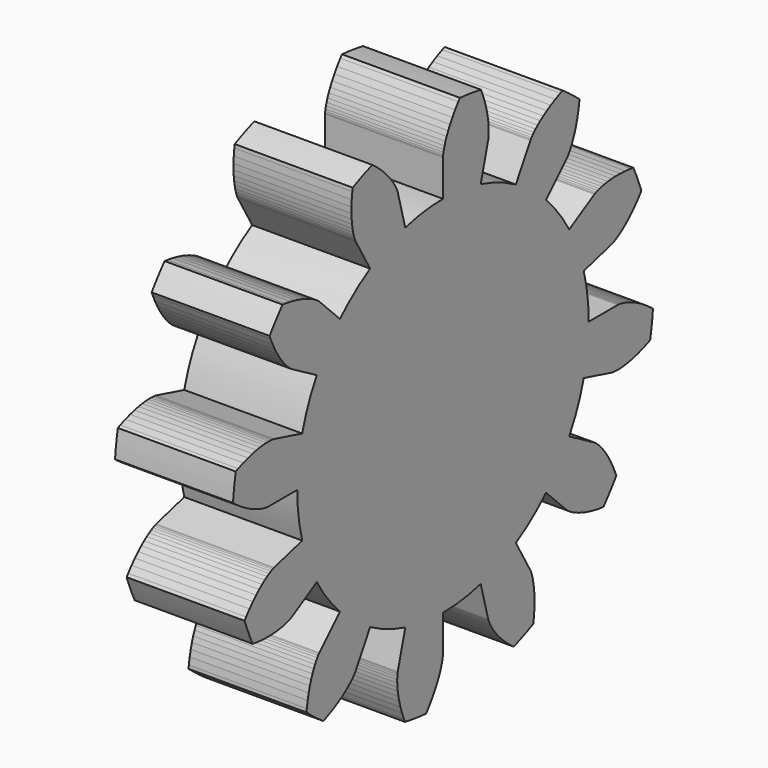
from build123d import *

# Parameters (mm, degrees)
F2_DEPTH = 4.9784


# Not quite as in the source:
# - a variable given as a bare number and used for a length is read in inches; the dataset says mm whatever the document's units were
# - a feature names something its author has since deleted; it is built from what else it names


with BuildPart() as f2:
    # F1 (on Right) → F2 (new body)
    with BuildSketch(Plane.YZ):
        with BuildLine():
            ThreePointArc((7.426291308, -1.9898687587), (7.6224883485, -1.0035196289), (7.6882625, 0))
            ThreePointArc((7.6882625, 0), (7.6224883485, 1.0035196289), (7.426291308, 1.9898687587))
            ThreePointArc((7.426291308, 1.9898687587), (7.1030283643, 2.9421706824), (6.658230636, 3.84413125))
            ThreePointArc((6.658230636, 3.84413125), (6.0995087354, 4.6803176661), (5.4364225493, 5.4364225493))
            ThreePointArc((5.4364225493, 5.4364225493), (4.6803176661, 6.0995087354), (3.84413125, 6.658230636))
            ThreePointArc((3.84413125, 6.658230636), (2.9421706824, 7.1030283643), (1.9898687587, 7.426291308))
            ThreePointArc((1.9898687587, 7.426291308), (1.0035196289, 7.6224883485), (0, 7.6882625))
            ThreePointArc((0, 7.6882625), (-1.0035196289, 7.6224883485), (-1.9898687587, 7.426291308))
            ThreePointArc((-1.9898687587, 7.426291308), (-2.9421706824, 7.1030283643), (-3.84413125, 6.658230636))
            ThreePointArc((-3.84413125, 6.658230636), (-4.6803176661, 6.0995087354), (-5.4364225493, 5.4364225493))
            ThreePointArc((-5.4364225493, 5.4364225493), (-6.0995087354, 4.6803176661), (-6.658230636, 3.84413125))
            ThreePointArc((-6.658230636, 3.84413125), (-7.1030283643, 2.9421706824), (-7.426291308, 1.9898687587))
            ThreePointArc((-7.426291308, 1.9898687587), (-7.6224883485, 1.0035196289), (-7.6882625, 0))
            ThreePointArc((-7.6882625, 0), (-7.6224883485, -1.0035196289), (-7.426291308, -1.9898687587))
            ThreePointArc((-7.426291308, -1.9898687587), (-7.1030283643, -2.9421706824), (-6.658230636, -3.84413125))
            ThreePointArc((-6.658230636, -3.84413125), (-6.0995087354, -4.6803176661), (-5.4364225493, -5.4364225493))
            ThreePointArc((-5.4364225493, -5.4364225493), (-4.6803176661, -6.0995087354), (-3.84413125, -6.658230636))
            ThreePointArc((-3.84413125, -6.658230636), (-2.9421706824, -7.1030283643), (-1.9898687587, -7.426291308))
            ThreePointArc((-1.9898687587, -7.426291308), (-1.0035196289, -7.6224883485), (0, -7.6882625))
            ThreePointArc((0, -7.6882625), (1.0035196289, -7.6224883485), (1.9898687587, -7.426291308))
            ThreePointArc((1.9898687587, -7.426291308), (2.9421706824, -7.1030283643), (3.84413125, -6.658230636))
            ThreePointArc((3.84413125, -6.658230636), (4.6803176661, -6.0995087354), (5.4364225493, -5.4364225493))
            ThreePointArc((5.4364225493, -5.4364225493), (6.0995087354, -4.6803176661), (6.658230636, -3.84413125))
            ThreePointArc((6.658230636, -3.84413125), (7.1030283643, -2.9421706824), (7.426291308, -1.9898687587))
        make_face()
        with BuildLine():
            Line((-7.9861452975, -4.6108031373), (-6.658230636, -3.84413125))
            ThreePointArc((-6.658230636, -3.84413125), (-7.1030283643, -2.9421706824), (-7.426291308, -1.9898687587))
            Line((-7.426291308, -1.9898687587), (-8.9073876605, -2.3867273303))
            Line((-8.9073876605, -2.3867273303), (-8.9184155168, -2.3900799169))
            Line((-8.9184155168, -2.3900799169), (-8.9510185414, -2.4015972974))
            Line((-8.9510185414, -2.4015972974), (-9.0043537789, -2.4234254288))
            Line((-9.0043537789, -2.4234254288), (-9.0774187142, -2.4576437216))
            Line((-9.0774187142, -2.4576437216), (-9.1690559502, -2.506254508))
            Line((-9.1690559502, -2.506254508), (-9.2779585375, -2.5711728191))
            Line((-9.2779585375, -2.5711728191), (-9.4026759353, -2.6542165076))
            Line((-9.4026759353, -2.6542165076), (-9.5416205821, -2.7570967551))
            Line((-9.5416205821, -2.7570967551), (-9.6930750526, -2.8814089993))
            Line((-9.6930750526, -2.8814089993), (-9.8551997753, -3.0286243154))
            Line((-9.8551997753, -3.0286243154), (-10.026041282, -3.2000812859))
            Line((-10.026041282, -3.2000812859), (-10.2035409604, -3.3969783891))
            Line((-10.2035409604, -3.3969783891), (-10.3855442775, -3.6203669371))
            Line((-10.3855442775, -3.6203669371), (-10.4672422557, -3.7315540743))
            ThreePointArc((-10.4672422557, -3.7315540743), (-10.266611305, -4.2525696422), (-10.0400651697, -4.762850789))
            Line((-10.0400651697, -4.762850789), (-9.9036747965, -4.7837027733))
            Line((-9.9036747965, -4.7837027733), (-9.6170194597, -4.8129665507))
            Line((-9.6170194597, -4.8129665507), (-9.3522809566, -4.8266826013))
            Line((-9.3522809566, -4.8266826013), (-9.1102393822, -4.8271177999))
            Line((-9.1102393822, -4.8271177999), (-8.891502943, -4.8165752574))
            Line((-8.891502943, -4.8165752574), (-8.696506429, -4.7973828052))
            Line((-8.696506429, -4.7973828052), (-8.5255104064, -4.7718814239))
            Line((-8.5255104064, -4.7718814239), (-8.3786011334, -4.7424136615))
            Line((-8.3786011334, -4.7424136615), (-8.2556911974, -4.7113120815))
            Line((-8.2556911974, -4.7113120815), (-8.1565208698, -4.6808877872))
            Line((-8.1565208698, -4.6808877872), (-8.0806601717, -4.6534190629))
            Line((-8.0806601717, -4.6534190629), (-8.0275116438, -4.6311401745))
            Line((-8.0275116438, -4.6311401745), (-7.9963138062, -4.6162303726))
            Line((-7.9963138062, -4.6162303726), (-7.9861452975, -4.6108031373))
        make_face()
        with BuildLine():
            Line((-4.6108031373, -7.9861452975), (-3.84413125, -6.658230636))
            ThreePointArc((-3.84413125, -6.658230636), (-4.6803176661, -6.0995087354), (-5.4364225493, -5.4364225493))
            Line((-5.4364225493, -5.4364225493), (-6.5206603302, -6.5206603302))
            Line((-6.5206603302, -6.5206603302), (-6.5285344406, -6.5290776835))
            Line((-6.5285344406, -6.5290776835), (-6.5510107979, -6.5553535399))
            Line((-6.5510107979, -6.5553535399), (-6.5862864028, -6.600924875))
            Line((-6.5862864028, -6.600924875), (-6.6324533465, -6.6670912534))
            Line((-6.6324533465, -6.6670912534), (-6.6875081276, -6.7550080474))
            Line((-6.6875081276, -6.7550080474), (-6.7493613792, -6.8656802476))
            Line((-6.7493613792, -6.8656802476), (-6.8158479698, -6.9999568903))
            Line((-6.8158479698, -6.9999568903), (-6.8847374398, -7.1585261217))
            Line((-6.8847374398, -7.1585261217), (-6.9537447366, -7.3419109184))
            Line((-6.9537447366, -7.3419109184), (-7.020541207, -7.5504654833))
            Line((-7.020541207, -7.5504654833), (-7.0827658066, -7.7843723288))
            Line((-7.0827658066, -7.7843723288), (-7.1380364857, -8.0436400613))
            Line((-7.1380364857, -8.0436400613), (-7.1839617079, -8.3281018773))
            Line((-7.1839617079, -8.3281018773), (-7.1991206639, -8.4652417518))
            ThreePointArc((-7.1991206639, -8.4652417518), (-6.7648613799, -8.816138994), (-6.3135260981, -9.1447823626))
            Line((-6.3135260981, -9.1447823626), (-6.184982578, -9.0946455241))
            Line((-6.184982578, -9.0946455241), (-5.9220998854, -8.9766610303))
            Line((-5.9220998854, -8.9766610303), (-5.685971591, -8.856170227))
            Line((-5.685971591, -8.856170227), (-5.4761398396, -8.7355263329))
            Line((-5.4761398396, -8.7355263329), (-5.2919797978, -8.6170280037))
            Line((-5.2919797978, -8.6170280037), (-5.1327040891, -8.5029085955))
            Line((-5.1327040891, -8.5029085955), (-4.9973678802, -8.3953257402))
            Line((-4.9973678802, -8.3953257402), (-4.884874599, -8.2963512728))
            Line((-4.884874599, -8.2963512728), (-4.7939822621, -8.2079615464))
            Line((-4.7939822621, -8.2079615464), (-4.7233103861, -8.1320281709))
            Line((-4.7233103861, -8.1320281709), (-4.6713474566, -8.0703092087))
            Line((-4.6713474566, -8.0703092087), (-4.6364589254, -8.0244408615))
            Line((-4.6364589254, -8.0244408615), (-4.6168957065, -7.9959296755))
            Line((-4.6168957065, -7.9959296755), (-4.6108031373, -7.9861452975))
        make_face()
        with BuildLine():
            Line((0, -9.2216062746), (0, -7.6882625))
            ThreePointArc((0, -7.6882625), (-1.0035196289, -7.6224883485), (-1.9898687587, -7.426291308))
            Line((-1.9898687587, -7.426291308), (-2.3867273303, -8.9073876605))
            Line((-2.3867273303, -8.9073876605), (-2.3893378333, -8.9186143575))
            Line((-2.3893378333, -8.9186143575), (-2.3956650015, -8.9526080953))
            Line((-2.3956650015, -8.9526080953), (-2.4034289039, -9.0097118316))
            Line((-2.4034289039, -9.0097118316), (-2.4103274608, -9.0900970681))
            Line((-2.4103274608, -9.0900970681), (-2.4140479028, -9.1937626356))
            Line((-2.4140479028, -9.1937626356), (-2.4122782899, -9.3205341983))
            Line((-2.4122782899, -9.3205341983), (-2.402719045, -9.4700644773))
            Line((-2.402719045, -9.4700644773), (-2.3830944604, -9.6418341949))
            Line((-2.3830944604, -9.6418341949), (-2.3511641342, -9.835153736))
            Line((-2.3511641342, -9.835153736), (-2.3047342919, -10.0491655225))
            Line((-2.3047342919, -10.0491655225), (-2.2416689532, -10.2828470925))
            Line((-2.2416689532, -10.2828470925), (-2.1599008991, -10.5350148748))
            Line((-2.1599008991, -10.5350148748), (-2.0574424002, -10.804328645))
            Line((-2.0574424002, -10.804328645), (-2.0020005039, -10.9306747382))
            ThreePointArc((-2.0020005039, -10.9306747382), (-1.450472311, -11.017431022), (-0.8952828071, -11.0763768871))
            Line((-0.8952828071, -11.0763768871), (-0.8090292724, -10.9686853513))
            Line((-0.8090292724, -10.9686853513), (-0.6403584294, -10.7350664361))
            Line((-0.6403584294, -10.7350664361), (-0.4961107295, -10.5126541924))
            Line((-0.4961107295, -10.5126541924), (-0.3747130493, -10.3032576395))
            Line((-0.3747130493, -10.3032576395), (-0.2744749393, -10.1085550552))
            Line((-0.2744749393, -10.1085550552), (-0.1935978336, -9.9300868943))
            Line((-0.1935978336, -9.9300868943), (-0.1301846662, -9.7692493041))
            Line((-0.1301846662, -9.7692493041), (-0.0822498606, -9.6272882604))
            Line((-0.0822498606, -9.6272882604), (-0.047729651, -9.5052943435))
            Line((-0.047729651, -9.5052943435), (-0.0244926989, -9.4041981733))
            Line((-0.0244926989, -9.4041981733), (-0.010350963, -9.3247665195))
            Line((-0.010350963, -9.3247665195), (-0.0030707823, -9.2675990999))
            Line((-0.0030707823, -9.2675990999), (-0.0003841307, -9.2331260791))
            Line((-0.0003841307, -9.2331260791), (0, -9.2216062746))
        make_face()
        with BuildLine():
            Line((4.6108031373, -7.9861452975), (3.84413125, -6.658230636))
            ThreePointArc((3.84413125, -6.658230636), (2.9421706824, -7.1030283643), (1.9898687587, -7.426291308))
            Line((1.9898687587, -7.426291308), (2.3867273303, -8.9073876605))
            Line((2.3867273303, -8.9073876605), (2.3900799169, -8.9184155168))
            Line((2.3900799169, -8.9184155168), (2.4015972974, -8.9510185414))
            Line((2.4015972974, -8.9510185414), (2.4234254288, -9.0043537789))
            Line((2.4234254288, -9.0043537789), (2.4576437216, -9.0774187142))
            Line((2.4576437216, -9.0774187142), (2.506254508, -9.1690559502))
            Line((2.506254508, -9.1690559502), (2.5711728191, -9.2779585375))
            Line((2.5711728191, -9.2779585375), (2.6542165076, -9.4026759353))
            Line((2.6542165076, -9.4026759353), (2.7570967551, -9.5416205821))
            Line((2.7570967551, -9.5416205821), (2.8814089993, -9.6930750526))
            Line((2.8814089993, -9.6930750526), (3.0286243154, -9.8551997753))
            Line((3.0286243154, -9.8551997753), (3.2000812859, -10.026041282))
            Line((3.2000812859, -10.026041282), (3.3969783891, -10.2035409604))
            Line((3.3969783891, -10.2035409604), (3.6203669371, -10.3855442775))
            Line((3.6203669371, -10.3855442775), (3.7315540743, -10.4672422557))
            ThreePointArc((3.7315540743, -10.4672422557), (4.2525696422, -10.266611305), (4.762850789, -10.0400651697))
            Line((4.762850789, -10.0400651697), (4.7837027733, -9.9036747965))
            Line((4.7837027733, -9.9036747965), (4.8129665507, -9.6170194597))
            Line((4.8129665507, -9.6170194597), (4.8266826013, -9.3522809566))
            Line((4.8266826013, -9.3522809566), (4.8271177999, -9.1102393822))
            Line((4.8271177999, -9.1102393822), (4.8165752574, -8.891502943))
            Line((4.8165752574, -8.891502943), (4.7973828052, -8.696506429))
            Line((4.7973828052, -8.696506429), (4.7718814239, -8.5255104064))
            Line((4.7718814239, -8.5255104064), (4.7424136615, -8.3786011334))
            Line((4.7424136615, -8.3786011334), (4.7113120815, -8.2556911974))
            Line((4.7113120815, -8.2556911974), (4.6808877872, -8.1565208698))
            Line((4.6808877872, -8.1565208698), (4.6534190629, -8.0806601717))
            Line((4.6534190629, -8.0806601717), (4.6311401745, -8.0275116438))
            Line((4.6311401745, -8.0275116438), (4.6162303726, -7.9963138062))
            Line((4.6162303726, -7.9963138062), (4.6108031373, -7.9861452975))
        make_face()
        with BuildLine():
            Line((7.9861452975, -4.6108031373), (6.658230636, -3.84413125))
            ThreePointArc((6.658230636, -3.84413125), (6.0995087354, -4.6803176661), (5.4364225493, -5.4364225493))
            Line((5.4364225493, -5.4364225493), (6.5206603302, -6.5206603302))
            Line((6.5206603302, -6.5206603302), (6.5290776835, -6.5285344406))
            Line((6.5290776835, -6.5285344406), (6.5553535399, -6.5510107979))
            Line((6.5553535399, -6.5510107979), (6.600924875, -6.5862864028))
            Line((6.600924875, -6.5862864028), (6.6670912534, -6.6324533465))
            Line((6.6670912534, -6.6324533465), (6.7550080474, -6.6875081276))
            Line((6.7550080474, -6.6875081276), (6.8656802476, -6.7493613792))
            Line((6.8656802476, -6.7493613792), (6.9999568903, -6.8158479698))
            Line((6.9999568903, -6.8158479698), (7.1585261217, -6.8847374398))
            Line((7.1585261217, -6.8847374398), (7.3419109184, -6.9537447366))
            Line((7.3419109184, -6.9537447366), (7.5504654833, -7.020541207))
            Line((7.5504654833, -7.020541207), (7.7843723288, -7.0827658066))
            Line((7.7843723288, -7.0827658066), (8.0436400613, -7.1380364857))
            Line((8.0436400613, -7.1380364857), (8.3281018773, -7.1839617079))
            Line((8.3281018773, -7.1839617079), (8.4652417518, -7.1991206639))
            ThreePointArc((8.4652417518, -7.1991206639), (8.816138994, -6.7648613799), (9.1447823626, -6.3135260981))
            Line((9.1447823626, -6.3135260981), (9.0946455241, -6.184982578))
            Line((9.0946455241, -6.184982578), (8.9766610303, -5.9220998854))
            Line((8.9766610303, -5.9220998854), (8.856170227, -5.685971591))
            Line((8.856170227, -5.685971591), (8.7355263329, -5.4761398396))
            Line((8.7355263329, -5.4761398396), (8.6170280037, -5.2919797978))
            Line((8.6170280037, -5.2919797978), (8.5029085955, -5.1327040891))
            Line((8.5029085955, -5.1327040891), (8.3953257402, -4.9973678802))
            Line((8.3953257402, -4.9973678802), (8.2963512728, -4.884874599))
            Line((8.2963512728, -4.884874599), (8.2079615464, -4.7939822621))
            Line((8.2079615464, -4.7939822621), (8.1320281709, -4.7233103861))
            Line((8.1320281709, -4.7233103861), (8.0703092087, -4.6713474566))
            Line((8.0703092087, -4.6713474566), (8.0244408615, -4.6364589254))
            Line((8.0244408615, -4.6364589254), (7.9959296755, -4.6168957065))
            Line((7.9959296755, -4.6168957065), (7.9861452975, -4.6108031373))
        make_face()
        with BuildLine():
            Line((9.2216062746, 0), (7.6882625, 0))
            ThreePointArc((7.6882625, 0), (7.6224883485, -1.0035196289), (7.426291308, -1.9898687587))
            Line((7.426291308, -1.9898687587), (8.9073876605, -2.3867273303))
            Line((8.9073876605, -2.3867273303), (8.9186143575, -2.3893378333))
            Line((8.9186143575, -2.3893378333), (8.9526080953, -2.3956650015))
            Line((8.9526080953, -2.3956650015), (9.0097118316, -2.4034289039))
            Line((9.0097118316, -2.4034289039), (9.0900970681, -2.4103274608))
            Line((9.0900970681, -2.4103274608), (9.1937626356, -2.4140479028))
            Line((9.1937626356, -2.4140479028), (9.3205341983, -2.4122782899))
            Line((9.3205341983, -2.4122782899), (9.4700644773, -2.402719045))
            Line((9.4700644773, -2.402719045), (9.6418341949, -2.3830944604))
            Line((9.6418341949, -2.3830944604), (9.835153736, -2.3511641342))
            Line((9.835153736, -2.3511641342), (10.0491655225, -2.3047342919))
            Line((10.0491655225, -2.3047342919), (10.2828470925, -2.2416689532))
            Line((10.2828470925, -2.2416689532), (10.5350148748, -2.1599008991))
            Line((10.5350148748, -2.1599008991), (10.804328645, -2.0574424002))
            Line((10.804328645, -2.0574424002), (10.9306747382, -2.0020005039))
            ThreePointArc((10.9306747382, -2.0020005039), (11.017431022, -1.450472311), (11.0763768871, -0.8952828071))
            Line((11.0763768871, -0.8952828071), (10.9686853513, -0.8090292724))
            Line((10.9686853513, -0.8090292724), (10.7350664361, -0.6403584294))
            Line((10.7350664361, -0.6403584294), (10.5126541924, -0.4961107295))
            Line((10.5126541924, -0.4961107295), (10.3032576395, -0.3747130493))
            Line((10.3032576395, -0.3747130493), (10.1085550552, -0.2744749393))
            Line((10.1085550552, -0.2744749393), (9.9300868943, -0.1935978336))
            Line((9.9300868943, -0.1935978336), (9.7692493041, -0.1301846662))
            Line((9.7692493041, -0.1301846662), (9.6272882604, -0.0822498606))
            Line((9.6272882604, -0.0822498606), (9.5052943435, -0.047729651))
            Line((9.5052943435, -0.047729651), (9.4041981733, -0.0244926989))
            Line((9.4041981733, -0.0244926989), (9.3247665195, -0.010350963))
            Line((9.3247665195, -0.010350963), (9.2675990999, -0.0030707823))
            Line((9.2675990999, -0.0030707823), (9.2331260791, -0.0003841307))
            Line((9.2331260791, -0.0003841307), (9.2216062746, 0))
        make_face()
        with BuildLine():
            ThreePointArc((6.658230636, 3.84413125), (7.1030283643, 2.9421706824), (7.426291308, 1.9898687587))
            Line((7.426291308, 1.9898687587), (8.9073876605, 2.3867273303))
            Line((8.9073876605, 2.3867273303), (8.9184155168, 2.3900799169))
            Line((8.9184155168, 2.3900799169), (8.9510185414, 2.4015972974))
            Line((8.9510185414, 2.4015972974), (9.0043537789, 2.4234254288))
            Line((9.0043537789, 2.4234254288), (9.0774187142, 2.4576437216))
            Line((9.0774187142, 2.4576437216), (9.1690559502, 2.506254508))
            Line((9.1690559502, 2.506254508), (9.2779585375, 2.5711728191))
            Line((9.2779585375, 2.5711728191), (9.4026759353, 2.6542165076))
            Line((9.4026759353, 2.6542165076), (9.5416205821, 2.7570967551))
            Line((9.5416205821, 2.7570967551), (9.6930750526, 2.8814089993))
            Line((9.6930750526, 2.8814089993), (9.8551997753, 3.0286243154))
            Line((9.8551997753, 3.0286243154), (10.026041282, 3.2000812859))
            Line((10.026041282, 3.2000812859), (10.2035409604, 3.3969783891))
            Line((10.2035409604, 3.3969783891), (10.3855442775, 3.6203669371))
            Line((10.3855442775, 3.6203669371), (10.4672422557, 3.7315540743))
            ThreePointArc((10.4672422557, 3.7315540743), (10.266611305, 4.2525696422), (10.0400651697, 4.762850789))
            Line((10.0400651697, 4.762850789), (9.9036747965, 4.7837027733))
            Line((9.9036747965, 4.7837027733), (9.6170194597, 4.8129665507))
            Line((9.6170194597, 4.8129665507), (9.3522809566, 4.8266826013))
            Line((9.3522809566, 4.8266826013), (9.1102393822, 4.8271177999))
            Line((9.1102393822, 4.8271177999), (8.891502943, 4.8165752574))
            Line((8.891502943, 4.8165752574), (8.696506429, 4.7973828052))
            Line((8.696506429, 4.7973828052), (8.5255104064, 4.7718814239))
            Line((8.5255104064, 4.7718814239), (8.3786011334, 4.7424136615))
            Line((8.3786011334, 4.7424136615), (8.2556911974, 4.7113120815))
            Line((8.2556911974, 4.7113120815), (8.1565208698, 4.6808877872))
            Line((8.1565208698, 4.6808877872), (8.0806601717, 4.6534190629))
            Line((8.0806601717, 4.6534190629), (8.0275116438, 4.6311401745))
            Line((8.0275116438, 4.6311401745), (7.9963138062, 4.6162303726))
            Line((7.9963138062, 4.6162303726), (7.9861452975, 4.6108031373))
            Line((7.9861452975, 4.6108031373), (6.658230636, 3.84413125))
        make_face()
        with BuildLine():
            ThreePointArc((3.84413125, 6.658230636), (4.6803176661, 6.0995087354), (5.4364225493, 5.4364225493))
            Line((5.4364225493, 5.4364225493), (6.5206603302, 6.5206603302))
            Line((6.5206603302, 6.5206603302), (6.5285344406, 6.5290776835))
            Line((6.5285344406, 6.5290776835), (6.5510107979, 6.5553535399))
            Line((6.5510107979, 6.5553535399), (6.5862864028, 6.600924875))
            Line((6.5862864028, 6.600924875), (6.6324533465, 6.6670912534))
            Line((6.6324533465, 6.6670912534), (6.6875081276, 6.7550080474))
            Line((6.6875081276, 6.7550080474), (6.7493613792, 6.8656802476))
            Line((6.7493613792, 6.8656802476), (6.8158479698, 6.9999568903))
            Line((6.8158479698, 6.9999568903), (6.8847374398, 7.1585261217))
            Line((6.8847374398, 7.1585261217), (6.9537447366, 7.3419109184))
            Line((6.9537447366, 7.3419109184), (7.020541207, 7.5504654833))
            Line((7.020541207, 7.5504654833), (7.0827658066, 7.7843723288))
            Line((7.0827658066, 7.7843723288), (7.1380364857, 8.0436400613))
            Line((7.1380364857, 8.0436400613), (7.1839617079, 8.3281018773))
            Line((7.1839617079, 8.3281018773), (7.1991206639, 8.4652417518))
            ThreePointArc((7.1991206639, 8.4652417518), (6.7648613799, 8.816138994), (6.3135260981, 9.1447823626))
            Line((6.3135260981, 9.1447823626), (6.184982578, 9.0946455241))
            Line((6.184982578, 9.0946455241), (5.9220998854, 8.9766610303))
            Line((5.9220998854, 8.9766610303), (5.685971591, 8.856170227))
            Line((5.685971591, 8.856170227), (5.4761398396, 8.7355263329))
            Line((5.4761398396, 8.7355263329), (5.2919797978, 8.6170280037))
            Line((5.2919797978, 8.6170280037), (5.1327040891, 8.5029085955))
            Line((5.1327040891, 8.5029085955), (4.9973678802, 8.3953257402))
            Line((4.9973678802, 8.3953257402), (4.884874599, 8.2963512728))
            Line((4.884874599, 8.2963512728), (4.7939822621, 8.2079615464))
            Line((4.7939822621, 8.2079615464), (4.7233103861, 8.1320281709))
            Line((4.7233103861, 8.1320281709), (4.6713474566, 8.0703092087))
            Line((4.6713474566, 8.0703092087), (4.6364589254, 8.0244408615))
            Line((4.6364589254, 8.0244408615), (4.6168957065, 7.9959296755))
            Line((4.6168957065, 7.9959296755), (4.6108031373, 7.9861452975))
            Line((4.6108031373, 7.9861452975), (3.84413125, 6.658230636))
        make_face()
        with BuildLine():
            ThreePointArc((0, 7.6882625), (1.0035196289, 7.6224883485), (1.9898687587, 7.426291308))
            Line((1.9898687587, 7.426291308), (2.3867273303, 8.9073876605))
            Line((2.3867273303, 8.9073876605), (2.3893378333, 8.9186143575))
            Line((2.3893378333, 8.9186143575), (2.3956650015, 8.9526080953))
            Line((2.3956650015, 8.9526080953), (2.4034289039, 9.0097118316))
            Line((2.4034289039, 9.0097118316), (2.4103274608, 9.0900970681))
            Line((2.4103274608, 9.0900970681), (2.4140479028, 9.1937626356))
            Line((2.4140479028, 9.1937626356), (2.4122782899, 9.3205341983))
            Line((2.4122782899, 9.3205341983), (2.402719045, 9.4700644773))
            Line((2.402719045, 9.4700644773), (2.3830944604, 9.6418341949))
            Line((2.3830944604, 9.6418341949), (2.3511641342, 9.835153736))
            Line((2.3511641342, 9.835153736), (2.3047342919, 10.0491655225))
            Line((2.3047342919, 10.0491655225), (2.2416689532, 10.2828470925))
            Line((2.2416689532, 10.2828470925), (2.1599008991, 10.5350148748))
            Line((2.1599008991, 10.5350148748), (2.0574424002, 10.804328645))
            Line((2.0574424002, 10.804328645), (2.0020005039, 10.9306747382))
            ThreePointArc((2.0020005039, 10.9306747382), (1.450472311, 11.017431022), (0.8952828071, 11.0763768871))
            Line((0.8952828071, 11.0763768871), (0.8090292724, 10.9686853513))
            Line((0.8090292724, 10.9686853513), (0.6403584294, 10.7350664361))
            Line((0.6403584294, 10.7350664361), (0.4961107295, 10.5126541924))
            Line((0.4961107295, 10.5126541924), (0.3747130493, 10.3032576395))
            Line((0.3747130493, 10.3032576395), (0.2744749393, 10.1085550552))
            Line((0.2744749393, 10.1085550552), (0.1935978336, 9.9300868943))
            Line((0.1935978336, 9.9300868943), (0.1301846662, 9.7692493041))
            Line((0.1301846662, 9.7692493041), (0.0822498606, 9.6272882604))
            Line((0.0822498606, 9.6272882604), (0.047729651, 9.5052943435))
            Line((0.047729651, 9.5052943435), (0.0244926989, 9.4041981733))
            Line((0.0244926989, 9.4041981733), (0.010350963, 9.3247665195))
            Line((0.010350963, 9.3247665195), (0.0030707823, 9.2675990999))
            Line((0.0030707823, 9.2675990999), (0.0003841307, 9.2331260791))
            Line((0.0003841307, 9.2331260791), (0, 9.2216062746))
            Line((0, 9.2216062746), (0, 7.6882625))
        make_face()
        with BuildLine():
            ThreePointArc((-3.84413125, 6.658230636), (-2.9421706824, 7.1030283643), (-1.9898687587, 7.426291308))
            Line((-1.9898687587, 7.426291308), (-2.3867273303, 8.9073876605))
            Line((-2.3867273303, 8.9073876605), (-2.3900799169, 8.9184155168))
            Line((-2.3900799169, 8.9184155168), (-2.4015972974, 8.9510185414))
            Line((-2.4015972974, 8.9510185414), (-2.4234254288, 9.0043537789))
            Line((-2.4234254288, 9.0043537789), (-2.4576437216, 9.0774187142))
            Line((-2.4576437216, 9.0774187142), (-2.506254508, 9.1690559502))
            Line((-2.506254508, 9.1690559502), (-2.5711728191, 9.2779585375))
            Line((-2.5711728191, 9.2779585375), (-2.6542165076, 9.4026759353))
            Line((-2.6542165076, 9.4026759353), (-2.7570967551, 9.5416205821))
            Line((-2.7570967551, 9.5416205821), (-2.8814089993, 9.6930750526))
            Line((-2.8814089993, 9.6930750526), (-3.0286243154, 9.8551997753))
            Line((-3.0286243154, 9.8551997753), (-3.2000812859, 10.026041282))
            Line((-3.2000812859, 10.026041282), (-3.3969783891, 10.2035409604))
            Line((-3.3969783891, 10.2035409604), (-3.6203669371, 10.3855442775))
            Line((-3.6203669371, 10.3855442775), (-3.7315540743, 10.4672422557))
            ThreePointArc((-3.7315540743, 10.4672422557), (-4.2525696422, 10.266611305), (-4.762850789, 10.0400651697))
            Line((-4.762850789, 10.0400651697), (-4.7837027733, 9.9036747965))
            Line((-4.7837027733, 9.9036747965), (-4.8129665507, 9.6170194597))
            Line((-4.8129665507, 9.6170194597), (-4.8266826013, 9.3522809566))
            Line((-4.8266826013, 9.3522809566), (-4.8271177999, 9.1102393822))
            Line((-4.8271177999, 9.1102393822), (-4.8165752574, 8.891502943))
            Line((-4.8165752574, 8.891502943), (-4.7973828052, 8.696506429))
            Line((-4.7973828052, 8.696506429), (-4.7718814239, 8.5255104064))
            Line((-4.7718814239, 8.5255104064), (-4.7424136615, 8.3786011334))
            Line((-4.7424136615, 8.3786011334), (-4.7113120815, 8.2556911974))
            Line((-4.7113120815, 8.2556911974), (-4.6808877872, 8.1565208698))
            Line((-4.6808877872, 8.1565208698), (-4.6534190629, 8.0806601717))
            Line((-4.6534190629, 8.0806601717), (-4.6311401745, 8.0275116438))
            Line((-4.6311401745, 8.0275116438), (-4.6162303726, 7.9963138062))
            Line((-4.6162303726, 7.9963138062), (-4.6108031373, 7.9861452975))
            Line((-4.6108031373, 7.9861452975), (-3.84413125, 6.658230636))
        make_face()
        with BuildLine():
            ThreePointArc((-6.658230636, 3.84413125), (-6.0995087354, 4.6803176661), (-5.4364225493, 5.4364225493))
            Line((-5.4364225493, 5.4364225493), (-6.5206603302, 6.5206603302))
            Line((-6.5206603302, 6.5206603302), (-6.5290776835, 6.5285344406))
            Line((-6.5290776835, 6.5285344406), (-6.5553535399, 6.5510107979))
            Line((-6.5553535399, 6.5510107979), (-6.600924875, 6.5862864028))
            Line((-6.600924875, 6.5862864028), (-6.6670912534, 6.6324533465))
            Line((-6.6670912534, 6.6324533465), (-6.7550080474, 6.6875081276))
            Line((-6.7550080474, 6.6875081276), (-6.8656802476, 6.7493613792))
            Line((-6.8656802476, 6.7493613792), (-6.9999568903, 6.8158479698))
            Line((-6.9999568903, 6.8158479698), (-7.1585261217, 6.8847374398))
            Line((-7.1585261217, 6.8847374398), (-7.3419109184, 6.9537447366))
            Line((-7.3419109184, 6.9537447366), (-7.5504654833, 7.020541207))
            Line((-7.5504654833, 7.020541207), (-7.7843723288, 7.0827658066))
            Line((-7.7843723288, 7.0827658066), (-8.0436400613, 7.1380364857))
            Line((-8.0436400613, 7.1380364857), (-8.3281018773, 7.1839617079))
            Line((-8.3281018773, 7.1839617079), (-8.4652417518, 7.1991206639))
            ThreePointArc((-8.4652417518, 7.1991206639), (-8.816138994, 6.7648613799), (-9.1447823626, 6.3135260981))
            Line((-9.1447823626, 6.3135260981), (-9.0946455241, 6.184982578))
            Line((-9.0946455241, 6.184982578), (-8.9766610303, 5.9220998854))
            Line((-8.9766610303, 5.9220998854), (-8.856170227, 5.685971591))
            Line((-8.856170227, 5.685971591), (-8.7355263329, 5.4761398396))
            Line((-8.7355263329, 5.4761398396), (-8.6170280037, 5.2919797978))
            Line((-8.6170280037, 5.2919797978), (-8.5029085955, 5.1327040891))
            Line((-8.5029085955, 5.1327040891), (-8.3953257402, 4.9973678802))
            Line((-8.3953257402, 4.9973678802), (-8.2963512728, 4.884874599))
            Line((-8.2963512728, 4.884874599), (-8.2079615464, 4.7939822621))
            Line((-8.2079615464, 4.7939822621), (-8.1320281709, 4.7233103861))
            Line((-8.1320281709, 4.7233103861), (-8.0703092087, 4.6713474566))
            Line((-8.0703092087, 4.6713474566), (-8.0244408615, 4.6364589254))
            Line((-8.0244408615, 4.6364589254), (-7.9959296755, 4.6168957065))
            Line((-7.9959296755, 4.6168957065), (-7.9861452975, 4.6108031373))
            Line((-7.9861452975, 4.6108031373), (-6.658230636, 3.84413125))
        make_face()
        with BuildLine():
            ThreePointArc((-7.6882625, 0), (-7.6224883485, 1.0035196289), (-7.426291308, 1.9898687587))
            Line((-7.426291308, 1.9898687587), (-8.9073876605, 2.3867273303))
            Line((-8.9073876605, 2.3867273303), (-8.9186143575, 2.3893378333))
            Line((-8.9186143575, 2.3893378333), (-8.9526080953, 2.3956650015))
            Line((-8.9526080953, 2.3956650015), (-9.0097118316, 2.4034289039))
            Line((-9.0097118316, 2.4034289039), (-9.0900970681, 2.4103274608))
            Line((-9.0900970681, 2.4103274608), (-9.1937626356, 2.4140479028))
            Line((-9.1937626356, 2.4140479028), (-9.3205341983, 2.4122782899))
            Line((-9.3205341983, 2.4122782899), (-9.4700644773, 2.402719045))
            Line((-9.4700644773, 2.402719045), (-9.6418341949, 2.3830944604))
            Line((-9.6418341949, 2.3830944604), (-9.835153736, 2.3511641342))
            Line((-9.835153736, 2.3511641342), (-10.0491655225, 2.3047342919))
            Line((-10.0491655225, 2.3047342919), (-10.2828470925, 2.2416689532))
            Line((-10.2828470925, 2.2416689532), (-10.5350148748, 2.1599008991))
            Line((-10.5350148748, 2.1599008991), (-10.804328645, 2.0574424002))
            Line((-10.804328645, 2.0574424002), (-10.9306747382, 2.0020005039))
            ThreePointArc((-10.9306747382, 2.0020005039), (-11.017431022, 1.450472311), (-11.0763768871, 0.8952828071))
            Line((-11.0763768871, 0.8952828071), (-10.9686853513, 0.8090292724))
            Line((-10.9686853513, 0.8090292724), (-10.7350664361, 0.6403584294))
            Line((-10.7350664361, 0.6403584294), (-10.5126541924, 0.4961107295))
            Line((-10.5126541924, 0.4961107295), (-10.3032576395, 0.3747130493))
            Line((-10.3032576395, 0.3747130493), (-10.1085550552, 0.2744749393))
            Line((-10.1085550552, 0.2744749393), (-9.9300868943, 0.1935978336))
            Line((-9.9300868943, 0.1935978336), (-9.7692493041, 0.1301846662))
            Line((-9.7692493041, 0.1301846662), (-9.6272882604, 0.0822498606))
            Line((-9.6272882604, 0.0822498606), (-9.5052943435, 0.047729651))
            Line((-9.5052943435, 0.047729651), (-9.4041981733, 0.0244926989))
            Line((-9.4041981733, 0.0244926989), (-9.3247665195, 0.010350963))
            Line((-9.3247665195, 0.010350963), (-9.2675990999, 0.0030707823))
            Line((-9.2675990999, 0.0030707823), (-9.2331260791, 0.0003841307))
            Line((-9.2331260791, 0.0003841307), (-9.2216062746, 0))
            Line((-9.2216062746, 0), (-7.6882625, 0))
        make_face()
    extrude(amount=F2_DEPTH)


solid = f2.part
